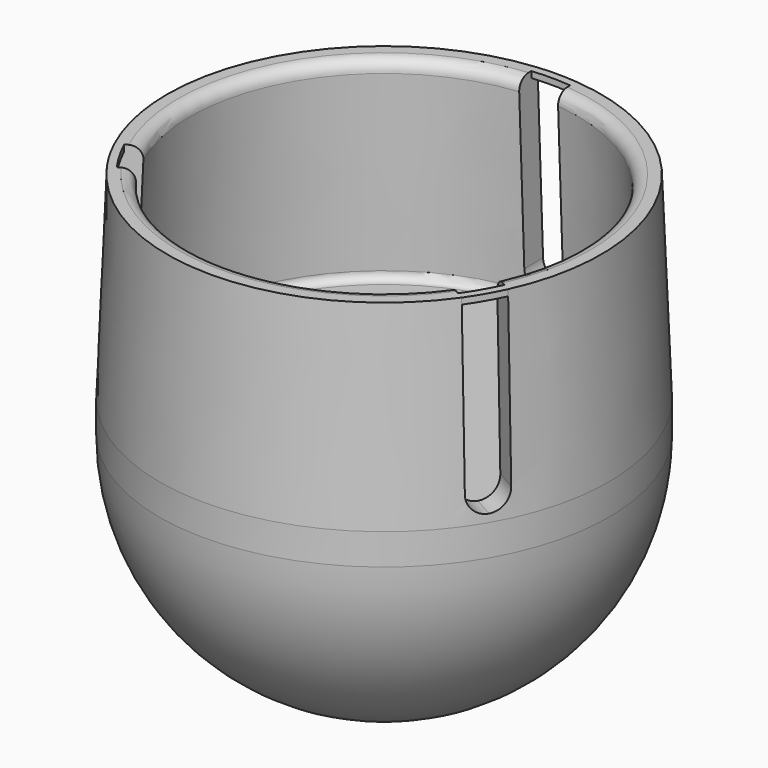
from build123d import *

# Parameters (mm, degrees)
F2_R      = 1
F3_R      = 1.5
F5_DEPTH  = 24.4
F6_F1_R   = 2.5
F6_F2_R   = 2.5
F6_F3_R   = 2.5
F6_F4_R   = 2.4999
F6_F5_R   = 2.4999
F6_F6_R   = 2.4999
F8_W      = 6.6521469513
F8_H      = 11.3077862186
F13_DEPTH = 6.192
F16_R     = 3.24
F17_DEPTH = 2.064
F7_R      = 27.892
F7_R_2    = 26.892
F18_DEPTH = 0.8


# Not quite as in the source:
# - a fillet or chamfer is up to 0.001 mm smaller than in the source, because OpenCascade refuses the exact size


with BuildPart() as f1:
    # F0 (on Front) → F1 (revolve)
    with BuildSketch(Plane.XZ):
        Polygon((0, -4), (0, 0), (-25.908, 0), (-24.892, 25.4), (-27.892, 25.4), (-28.908, 0), (-28.908, -4), align=None)
    revolve(axis=Axis((0, 0, -2), (0, 0, -1)))

    # F2
    f2_edges = [f1.edges().sort_by_distance(p)[0] for p in [
        (25.908, 0, 0),
    ]]
    fillet(f2_edges, radius=F2_R)

    # F3
    f3_edges = [f1.edges().sort_by_distance(p)[0] for p in [
        (24.892, 0, 25.4),
    ]]
    fillet(f3_edges, radius=F3_R)

    # F4 (on face) → F5 (cut)
    with BuildSketch(Plane.XY.offset(25.4)):
        Polygon((2.5, 32.8202601522), (-2.5, 32.8202601522), (-2.5, 1.443375673), (-1.25, 2.1650635095), (0, 0), (1.25, 2.1650635095), (2.5, 1.443375673), align=None)
        Polygon((-1.25, 2.1650635095), (-2.5, 1.443375673), (-2.5, 0), (0, 0), align=None)
        Polygon((-2.5, 0), (-2.5, 1.443375673), (-29.6731790506, -14.2450665666), (-27.1731790506, -18.5751935856), (0, -2.8867513459), (-1.25, -2.1650635095), (0, 0), align=None)
        Polygon((29.6731790506, -14.2450665666), (2.5, 1.443375673), (2.5, 0), (0, 0), (1.25, -2.1650635095), (0, -2.8867513459), (27.1731790506, -18.5751935856), align=None)
        Polygon((2.5, 0), (2.5, 1.443375673), (1.25, 2.1650635095), (0, 0), align=None)
        Polygon((1.25, -2.1650635095), (0, 0), (-1.25, -2.1650635095), (0, -2.8867513459), align=None)
    extrude(amount=-F5_DEPTH, mode=Mode.SUBTRACT)

    # F6: fillet of radius 2.5 on 6 edges, made by hand

    # F6_f1
    f6_f1_edges = [f1.edges().sort_by_distance(p)[0] for p in [
        (-22.351639831, -15.7914766192, 1),
    ]]
    fillet(f6_f1_edges, radius=F6_F1_R)

    # F6_f2
    f6_f2_edges = [f1.edges().sort_by_distance(p)[0] for p in [
        (2.5, 27.2528262195, 1),
    ]]
    fillet(f6_f2_edges, radius=F6_F2_R)

    # F6_f3
    f6_f3_edges = [f1.edges().sort_by_distance(p)[0] for p in [
        (22.351639831, -15.7914766192, 1),
    ]]
    fillet(f6_f3_edges, radius=F6_F3_R)

    # F6_f4 (radius 2.5 in the source; OpenCascade refuses exactly that, so slightly less here)
    f6_f4_edges = [f1.edges().sort_by_distance(p)[0] for p in [
        (-24.851639831, -11.4613496003, 1),
    ]]
    fillet(f6_f4_edges, radius=F6_F4_R)

    # F6_f5 (radius 2.5 in the source; OpenCascade refuses exactly that, so slightly less here)
    f6_f5_edges = [f1.edges().sort_by_distance(p)[0] for p in [
        (24.851639831, -11.4613496003, 1),
    ]]
    fillet(f6_f5_edges, radius=F6_F5_R)

    # F6_f6 (radius 2.5 in the source; OpenCascade refuses exactly that, so slightly less here)
    f6_f6_edges = [f1.edges().sort_by_distance(p)[0] for p in [
        (-2.5, 27.2528262195, 1),
    ]]
    fillet(f6_f6_edges, radius=F6_F6_R)

    # F8 (on Front) → F9 (revolve, cut)
    with BuildSketch(Plane.XZ):
        with Locations((-3.3260734756, 5.6538931093)):
            Rectangle(F8_W, F8_H)
        Polygon((0, -15.6807032946), (0, 0), (-6.6521469513, 0), (-3.24, -3.9252260535), (-3.24, -15.6807032946), (-3.175, -15.6807032946), align=None)
    revolve(axis=Axis((0, 0, -2.186458538), (0, 0, -1)), mode=Mode.SUBTRACT)

    # F7 (on face) → F18 (join)
    with BuildSketch(Plane.XY.offset(25.4)):
        Circle(F7_R)
        Circle(F7_R_2, mode=Mode.SUBTRACT)
    extrude(amount=-F18_DEPTH)


with BuildPart() as f11:
    # F10 (on Front) → F11 (revolve)
    with BuildSketch(Plane.XZ):
        with BuildLine():
            Line((0, -4), (-28.908, -4))
            ThreePointArc((-28.908, -4), (-24.4644892038, -19.40004), (-12.5, -30.0657335212))
            Line((-12.5, -30.0657335212), (0, -30.0657335212))
            Line((0, -30.0657335212), (0, -4))
        make_face()
    revolve(axis=Axis((0, 0, -17.0328667606), (0, 0, -1)))


with BuildPart() as f13:
    # F12 (on face) → F13 (new body)
    with BuildSketch(Plane.XY.offset(-4)):
        Polygon((3.2331615075, 5.6), (-3.2331615075, 5.6), (-6.4663230149, 0), (-3.2331615075, -5.6), (3.2331615075, -5.6), (6.4663230149, 0), align=None)
    extrude(amount=-F13_DEPTH)


with BuildPart() as f13_1:
    # F14: moved
    add(f13.part.moved(Location((0, 0, -2.064))))


with BuildPart() as f11_1:
    add(f11.part)

    # F15: cut F13
    add(f13_1.part, mode=Mode.SUBTRACT)

    # F16 (on face) → F17 (cut)
    with BuildSketch(Plane.XY.offset(-4)):
        Circle(F16_R)
    extrude(amount=-F17_DEPTH, mode=Mode.SUBTRACT)


solid = Compound([f1.part, f11_1.part])
